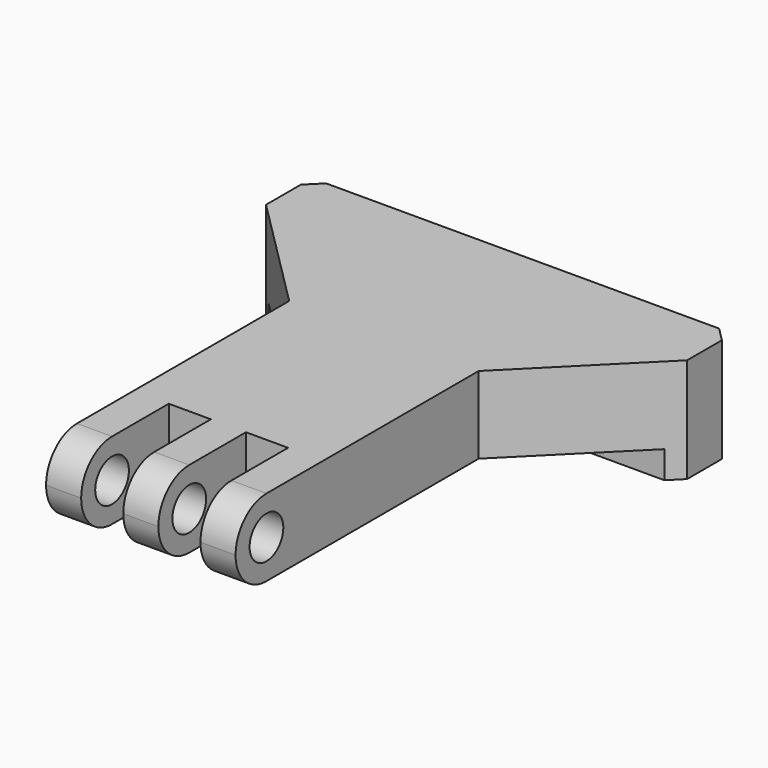
from build123d import *

# Parameters (mm, degrees)
F1_DEPTH = 2.75
F2_W     = 30
F2_H     = 5
F3_DEPTH = 1.95
F4_SIZE  = 8.24999
F5_SIZE  = 1
F6_R     = 2.74999
F8_D     = 3


# Not quite as in the source:
# - a fillet or chamfer is up to 0.001 mm smaller than in the source, because OpenCascade refuses the exact size


with BuildPart() as f1:
    # F0 (on Top) → F1 (new body, symmetric)
    with BuildSketch(Plane.XY):
        Polygon((-15, 17), (-15, 12), (-15, 4.65), (-6.75, 4.65), (-6.75, -17), (-4.25, -17), (-4.25, -9.2), (-1.25, -9.2), (-1.25, -17), (1.25, -17), (1.25, -9.2), (4.25, -9.2), (4.25, -17), (6.75, -17), (6.75, 4.65), (15, 4.65), (15, 12), (15, 17), align=None)
    extrude(amount=F1_DEPTH, both=True)

    # F2 (on face) → F3 (join)
    with BuildSketch(Plane(origin=(0, 0, -2.75), x_dir=(1, 0, 0), z_dir=(0, 0, -1))):
        with Locations((0, -14.5)):
            Rectangle(F2_W, F2_H)
    extrude(amount=F3_DEPTH)

    # F4 (size 8.25 in the source; OpenCascade refuses exactly that, so slightly less here)
    f4_edges = [f1.edges().sort_by_distance(p)[0] for p in [
        (-15, 4.65, 0),
        (15, 4.65, 0),
    ]]
    chamfer(f4_edges, length=F4_SIZE)

    # F5
    f5_edges = [f1.edges().sort_by_distance(p)[0] for p in [
        (15, 17, -0.975),
        (-15, 17, -0.975),
    ]]
    chamfer(f5_edges, length=F5_SIZE)

    # F6 (radius 2.75 in the source; OpenCascade refuses exactly that, so slightly less here)
    f6_edges = [f1.edges().sort_by_distance(p)[0] for p in [
        (5.5, -17, 2.75),
        (0, -17, 2.75),
        (-5.5, -17, 2.75),
        (5.5, -17, -2.75),
        (0, -17, -2.75),
        (-5.5, -17, -2.75),
    ]]
    fillet(f6_edges, radius=F6_R)

    # F8 (through all)
    with Locations(Plane.YZ.offset(6.75)):
        with Locations((-14.25, 0)):
            Hole(F8_D / 2)


solid = f1.part
